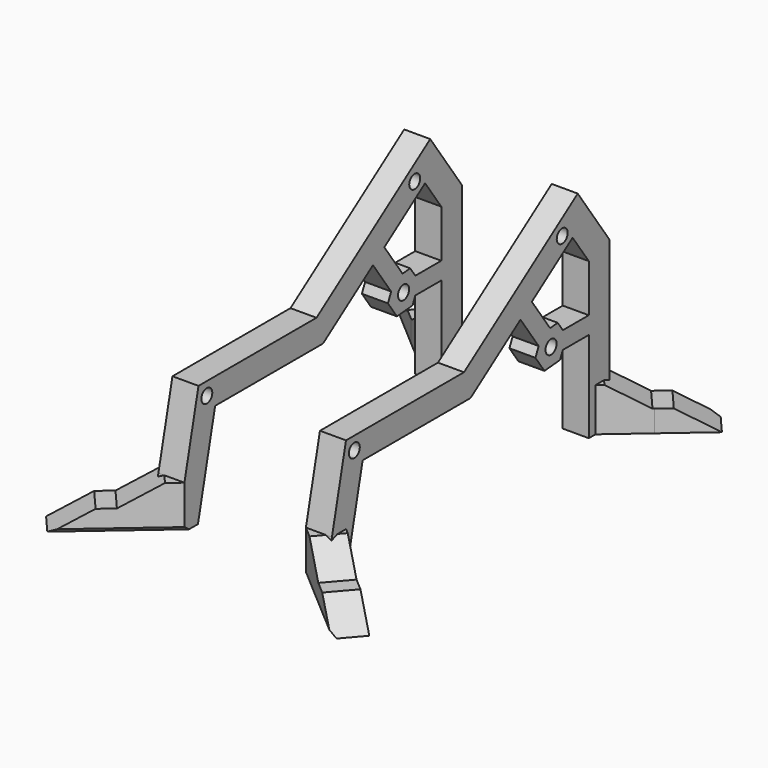
from build123d import *

# Parameters (mm, degrees)
F1_DEPTH     = 70
F2_DEPTH     = 10
F3_DEPTH     = 5
F4_R         = 1.6
F4_R_2       = 1.575
F5_DEPTH     = 25
F6_DEPTH     = 5
F7_SIZE      = 1
F8_T1_DEPTH  = 53.5675435836
F8_T6_DEPTH  = 53.5675435836
F8_T13_DEPTH = 53.5675435836
F8_T19_DEPTH = 53.5675435836
F8_T26_DEPTH = 53.5675435836
F8_T33_DEPTH = 53.5675435836
F9_T1_DEPTH  = 53.5675435836
F9_T6_DEPTH  = 53.5675435836
F9_T12_DEPTH = 53.5675435836
F9_T19_DEPTH = 53.5675435836
F9_T26_DEPTH = 53.5675435836
F9_T32_DEPTH = 53.5675435836


# Not quite as in the source:
# - a fillet or chamfer that OpenCascade refuses, or shapes differently, is made with other operations: its cross-section is extruded or revolved along the edge and cut away or added


with BuildPart() as f1:
    # F0 (on Top) → F1 (new body)
    with BuildSketch(Plane.XY):
        with BuildLine():
            Line((17.481584177, 40), (14, 40))
            Line((14, 40), (18.5698965916, 34.6975434805))
            Line((18.5698965916, 34.6975434805), (20, 35.9300712093))
            Line((20, 35.9300712093), (20, 38.5762325992))
            ThreePointArc((20, 38.5762325992), (18.1979669018, 38.327945742), (17.481584177, 40))
        make_face()
        with BuildLine():
            Line((20, 40), (17.481584177, 40))
            ThreePointArc((17.481584177, 40), (18.1979669018, 38.327945742), (20, 38.5762325992))
            Line((20, 38.5762325992), (20, 40))
        make_face()
        Polygon((18.5698965916, 34.6975434805), (14, 40), (14, 0), (14, -40), (18.5698965916, -34.6975434805), (20, -35.9300712093), (20, 0), (20, 35.9300712093), align=None)
        with BuildLine():
            Line((18.5698965916, -34.6975434805), (14, -40))
            Line((14, -40), (17.481584177, -40))
            ThreePointArc((17.481584177, -40), (18.1979669018, -38.327945742), (20, -38.5762325992))
            Line((20, -38.5762325992), (20, -35.9300712093))
            Line((20, -35.9300712093), (18.5698965916, -34.6975434805))
        make_face()
        with BuildLine():
            ThreePointArc((20, -38.5762325992), (18.1979669018, -38.327945742), (17.481584177, -40))
            Line((17.481584177, -40), (20, -40))
            Line((20, -40), (20, -38.5762325992))
        make_face()
    extrude(amount=F1_DEPTH)

    # F0 (on Top) → F2 (join)
    with BuildSketch(Plane.XY):
        with BuildLine():
            ThreePointArc((20.4361765556, 39.633720036), (19.1207184642, 41.1223248473), (17.481584177, 40))
            Line((17.481584177, 40), (20, 40))
            Line((20, 40), (20, 38.5762325992))
            ThreePointArc((20, 38.5762325992), (20.3228515656, 39.0617651281), (20.4361765556, 39.633720036))
        make_face()
        with BuildLine():
            Line((23.4686723563, 48.1605296279), (14, 40))
            Line((14, 40), (17.481584177, 40))
            ThreePointArc((17.481584177, 40), (19.1207184642, 41.1223248473), (20.4361765556, 39.633720036))
            ThreePointArc((20.4361765556, 39.633720036), (20.3228515656, 39.0617651281), (20, 38.5762325992))
            Line((20, 38.5762325992), (20, 35.9300712093))
            Line((20, 35.9300712093), (28.038568948, 42.8580731084))
            Line((28.038568948, 42.8580731084), (23.4686723563, 48.1605296279))
        make_face()
        with BuildLine():
            Line((17.481584177, -40), (14, -40))
            Line((14, -40), (23.4686723563, -48.1605296279))
            Line((23.4686723563, -48.1605296279), (28.038568948, -42.8580731084))
            Line((28.038568948, -42.8580731084), (20, -35.9300712093))
            Line((20, -35.9300712093), (20, -38.5762325992))
            ThreePointArc((20, -38.5762325992), (20.3228515656, -39.0617651281), (20.4361765556, -39.633720036))
            ThreePointArc((20.4361765556, -39.633720036), (19.1207184642, -41.1223248473), (17.481584177, -40))
        make_face()
        with BuildLine():
            Line((20, -40), (17.481584177, -40))
            ThreePointArc((17.481584177, -40), (19.1207184642, -41.1223248473), (20.4361765556, -39.633720036))
            ThreePointArc((20.4361765556, -39.633720036), (20.3228515656, -39.0617651281), (20, -38.5762325992))
            Line((20, -38.5762325992), (20, -40))
        make_face()
    extrude(amount=F2_DEPTH)

    # F0 (on Top) → F3 (join)
    with BuildSketch(Plane.XY):
        Polygon((32.9373447127, 56.3210592559), (23.4686723563, 48.1605296279), (28.038568948, 42.8580731084), (37.5072413043, 51.0186027363), align=None)
        Polygon((28.038568948, -42.8580731084), (23.4686723563, -48.1605296279), (32.9373447127, -56.3210592559), (37.5072413043, -51.0186027363), align=None)
    extrude(amount=F3_DEPTH)

    # F4 (on face) → F5 (cut)
    with BuildSketch(Plane(origin=(14, 0, 0), x_dir=(0, -1, 0), z_dir=(-1, 0, 0))):
        Polygon((-34, 0), (36.0994255375, 0), (31.1508810268, 22), (0.0593981216, 22), (-14.3160304975, 32.0657834841), (-19.5621121893, 24.5736023727), (-18.6246911161, 22.5632963938), (-21.2215746664, 18.8545623277), (-25.7318743586, 19.2491624199), (-26.5286701393, 20.9578964859), (-34, 20.9578964859), align=None)
        Polygon((-30.8148909167, 50.943057454), (1.9511908549, 28), (35.9511908549, 28), (40, 10), (40, 70), (-40, 70), (-40, 37.825362225), align=None)
        Polygon((-34, 24.9578964859), (-26.5211773832, 24.9578964859), (-25.0484069503, 27.0612306442), (-22.8387203665, 26.8679081181), (-17.5926386747, 34.3600892295), (-29.3414372691, 42.5866865702), (-34, 35.9335694917), align=None)
        with Locations((-23.1349908083, 22.9578964859)):
            Circle(F4_R)
        with Locations((-26.3438594686, 44.1500837642)):
            Circle(F4_R_2)
        with Locations((33.5510359408, 25)):
            Circle(F4_R_2)
    extrude(amount=-F5_DEPTH, mode=Mode.SUBTRACT)

    # F0 (on Top) → F6 (cut)
    with BuildSketch(Plane.XY):
        with BuildLine():
            Line((20, -40), (17.481584177, -40))
            ThreePointArc((17.481584177, -40), (19.1207184642, -41.1223248473), (20.4361765556, -39.633720036))
            ThreePointArc((20.4361765556, -39.633720036), (20.3228515656, -39.0617651281), (20, -38.5762325992))
            Line((20, -38.5762325992), (20, -40))
        make_face()
        with BuildLine():
            ThreePointArc((20, -38.5762325992), (18.1979669018, -38.327945742), (17.481584177, -40))
            Line((17.481584177, -40), (20, -40))
            Line((20, -40), (20, -38.5762325992))
        make_face()
        with BuildLine():
            ThreePointArc((20.4361765556, 39.633720036), (19.1207184642, 41.1223248473), (17.481584177, 40))
            Line((17.481584177, 40), (20, 40))
            Line((20, 40), (20, 38.5762325992))
            ThreePointArc((20, 38.5762325992), (20.3228515656, 39.0617651281), (20.4361765556, 39.633720036))
        make_face()
        with BuildLine():
            Line((20, 40), (17.481584177, 40))
            ThreePointArc((17.481584177, 40), (18.1979669018, 38.327945742), (20, 38.5762325992))
            Line((20, 38.5762325992), (20, 40))
        make_face()
    extrude(amount=F6_DEPTH, mode=Mode.SUBTRACT)

    # F7
    f7_edges = [f1.edges().sort_by_distance(p)[0] for p in [
        (23.468672, -48.16053, 0),
        (23.468672, 48.16053, 0),
    ]]
    chamfer(f7_edges, length=F7_SIZE)

    # F8: chamfer of 9 x 5.1961524227 on 2 edges, made by hand

    # F8_s2 → F8_t1 (cut)
    with BuildSketch(Plane(origin=(-29.0147501324, -33.6658495258, 0), x_dir=(0, 0, 1), z_dir=(0.6528423702, 0.7574937885, 0))):
        Polygon((-0.1961524227, 61.7186078485), (5, 52.7186078485), (5, 61.7186078485), align=None)
    extrude(amount=F8_T1_DEPTH, mode=Mode.SUBTRACT)


with BuildPart() as f8_tool4:
    # F8_s5 → F8_t6 (new body)
    with BuildSketch(Plane(origin=(-29.0147501324, -33.6658495258, 0), x_dir=(0, 0, 1), z_dir=(0.6528423702, 0.7574937885, 0))):
        Polygon((10, 40.2186078485), (4.8038475773, 49.2186078485), (10, 49.2186078485), align=None)
    extrude(amount=F8_T6_DEPTH)

    split(bisect_by=Plane(origin=(0, -40.2146679203, 9.0456397358), x_dir=(1, 0, 0), z_dir=(0, -0.9756235772, 0.219450759)), keep=Keep.TOP)

    split(bisect_by=Plane.YZ.offset(20), keep=Keep.BOTTOM)

    split(bisect_by=Plane.XY.offset(5), keep=Keep.TOP)


with BuildPart() as f1_1:
    add(f1.part)

    # F8_t3: cut F8_tool4
    add(f8_tool4.part, mode=Mode.SUBTRACT)


with BuildPart() as f8_tool11:
    # F8_s12 → F8_t13 (new body)
    with BuildSketch(Plane(origin=(-29.0147501324, -33.6658495258, 0), x_dir=(0, 0, 1), z_dir=(0.6528423702, 0.7574937885, 0))):
        Polygon((10, 40.2186078485), (4.8038475773, 49.2186078485), (10, 49.2186078485), align=None)
    extrude(amount=F8_T13_DEPTH)

    split(bisect_by=Plane.YZ.offset(20), keep=Keep.BOTTOM)

    split(bisect_by=Plane.XY.offset(5), keep=Keep.BOTTOM)


with BuildPart() as f1_2:
    add(f1_1.part)

    # F8_t10: cut F8_tool11
    add(f8_tool11.part, mode=Mode.SUBTRACT)


with BuildPart() as f8_tool17:
    # F8_s18 → F8_t19 (new body)
    with BuildSketch(Plane(origin=(-29.0147501324, -33.6658495258, 0), x_dir=(0, 0, 1), z_dir=(0.6528423702, 0.7574937885, 0))):
        Polygon((10, 40.2186078485), (4.8038475773, 49.2186078485), (10, 49.2186078485), align=None)
    extrude(amount=F8_T19_DEPTH)

    split(bisect_by=Plane(origin=(0, -40.2146679203, 9.0456397358), x_dir=(1, 0, 0), z_dir=(0, -0.9756235772, 0.219450759)), keep=Keep.TOP)

    split(bisect_by=Plane.YZ.offset(20), keep=Keep.TOP)

    split(bisect_by=Plane.XY.offset(5), keep=Keep.TOP)


with BuildPart() as f1_3:
    add(f1_2.part)

    # F8_t16: cut F8_tool17
    add(f8_tool17.part, mode=Mode.SUBTRACT)


with BuildPart() as f8_tool24:
    # F8_s25 → F8_t26 (new body)
    with BuildSketch(Plane(origin=(-29.0147501324, -33.6658495258, 0), x_dir=(0, 0, 1), z_dir=(0.6528423702, 0.7574937885, 0))):
        Polygon((10, 40.2186078485), (4.8038475773, 49.2186078485), (10, 49.2186078485), align=None)
    extrude(amount=F8_T26_DEPTH)

    split(bisect_by=Plane(origin=(0, -40.2146679203, 9.0456397358), x_dir=(1, 0, 0), z_dir=(0, 0.9756235772, -0.219450759)), keep=Keep.TOP)

    split(bisect_by=Plane.YZ.offset(20), keep=Keep.TOP)

    split(bisect_by=Plane.XY.offset(5), keep=Keep.TOP)


with BuildPart() as f1_4:
    add(f1_3.part)

    # F8_t23: cut F8_tool24
    add(f8_tool24.part, mode=Mode.SUBTRACT)


with BuildPart() as f8_tool31:
    # F8_s32 → F8_t33 (new body)
    with BuildSketch(Plane(origin=(-29.0147501324, -33.6658495258, 0), x_dir=(0, 0, 1), z_dir=(0.6528423702, 0.7574937885, 0))):
        Polygon((10, 40.2186078485), (4.8038475773, 49.2186078485), (10, 49.2186078485), align=None)
    extrude(amount=F8_T33_DEPTH)

    split(bisect_by=Plane(origin=(0, -40.2146679203, 9.0456397358), x_dir=(1, 0, 0), z_dir=(0, 0.9756235772, -0.219450759)), keep=Keep.TOP)

    split(bisect_by=Plane.XY.offset(5), keep=Keep.BOTTOM)


with BuildPart() as f1_5:
    add(f1_4.part)

    # F8_t30: cut F8_tool31
    add(f8_tool31.part, mode=Mode.SUBTRACT)

    # F9: chamfer of 9 x 5.1961524227 on 2 edges, made by hand

    # F9_s2 → F9_t1 (cut)
    with BuildSketch(Plane(origin=(5.9564119884, -6.9112320044, 0), x_dir=(0, 0, 1), z_dir=(-0.6528423702, 0.7574937885, 0))):
        Polygon((-0.1961524227, 61.7186078485), (5, 52.7186078485), (5, 61.7186078485), align=None)
    extrude(amount=F9_T1_DEPTH, mode=Mode.SUBTRACT)


with BuildPart() as f9_tool4:
    # F9_s5 → F9_t6 (new body)
    with BuildSketch(Plane(origin=(5.9564119884, -6.9112320044, 0), x_dir=(0, 0, 1), z_dir=(-0.6528423702, 0.7574937885, 0))):
        Polygon((4.8038475773, 49.2186078485), (10, 40.2186078485), (10, 49.2186078485), align=None)
    extrude(amount=F9_T6_DEPTH)

    split(bisect_by=Plane.XY.offset(5), keep=Keep.BOTTOM)

    split(bisect_by=Plane.XZ.offset(-40), keep=Keep.TOP)


with BuildPart() as f1_6:
    add(f1_5.part)

    # F9_t3: cut F9_tool4
    add(f9_tool4.part, mode=Mode.SUBTRACT)


with BuildPart() as f9_tool10:
    # F9_s11 → F9_t12 (new body)
    with BuildSketch(Plane(origin=(5.9564119884, -6.9112320044, 0), x_dir=(0, 0, 1), z_dir=(-0.6528423702, 0.7574937885, 0))):
        Polygon((4.8038475773, 49.2186078485), (10, 40.2186078485), (10, 49.2186078485), align=None)
    extrude(amount=F9_T12_DEPTH)

    split(bisect_by=Plane.YZ.offset(20), keep=Keep.TOP)

    split(bisect_by=Plane.XY.offset(5), keep=Keep.TOP)

    split(bisect_by=Plane.XZ.offset(-40), keep=Keep.TOP)


with BuildPart() as f1_7:
    add(f1_6.part)

    # F9_t9: cut F9_tool10
    add(f9_tool10.part, mode=Mode.SUBTRACT)


with BuildPart() as f9_tool17:
    # F9_s18 → F9_t19 (new body)
    with BuildSketch(Plane(origin=(5.9564119884, -6.9112320044, 0), x_dir=(0, 0, 1), z_dir=(-0.6528423702, 0.7574937885, 0))):
        Polygon((4.8038475773, 49.2186078485), (10, 40.2186078485), (10, 49.2186078485), align=None)
    extrude(amount=F9_T19_DEPTH)

    split(bisect_by=Plane.YZ.offset(20), keep=Keep.TOP)

    split(bisect_by=Plane.XY.offset(5), keep=Keep.TOP)

    split(bisect_by=Plane.XZ.offset(-40), keep=Keep.BOTTOM)


with BuildPart() as f1_8:
    add(f1_7.part)

    # F9_t16: cut F9_tool17
    add(f9_tool17.part, mode=Mode.SUBTRACT)


with BuildPart() as f9_tool24:
    # F9_s25 → F9_t26 (new body)
    with BuildSketch(Plane(origin=(5.9564119884, -6.9112320044, 0), x_dir=(0, 0, 1), z_dir=(-0.6528423702, 0.7574937885, 0))):
        Polygon((4.8038475773, 49.2186078485), (10, 40.2186078485), (10, 49.2186078485), align=None)
    extrude(amount=F9_T26_DEPTH)

    split(bisect_by=Plane.YZ.offset(20), keep=Keep.BOTTOM)

    split(bisect_by=Plane.XY.offset(5), keep=Keep.BOTTOM)


with BuildPart() as f1_9:
    add(f1_8.part)

    # F9_t23: cut F9_tool24
    add(f9_tool24.part, mode=Mode.SUBTRACT)


with BuildPart() as f9_tool30:
    # F9_s31 → F9_t32 (new body)
    with BuildSketch(Plane(origin=(5.9564119884, -6.9112320044, 0), x_dir=(0, 0, 1), z_dir=(-0.6528423702, 0.7574937885, 0))):
        Polygon((4.8038475773, 49.2186078485), (10, 40.2186078485), (10, 49.2186078485), align=None)
    extrude(amount=F9_T32_DEPTH)

    split(bisect_by=Plane.YZ.offset(20), keep=Keep.BOTTOM)

    split(bisect_by=Plane.XY.offset(5), keep=Keep.TOP)

    split(bisect_by=Plane.XZ.offset(-40), keep=Keep.BOTTOM)


with BuildPart() as f1_10:
    add(f1_9.part)

    # F9_t29: cut F9_tool30
    add(f9_tool30.part, mode=Mode.SUBTRACT)


with BuildPart() as f10_1:
    # F10: instance of F1
    add(f1_10.part.mirror(Plane.YZ))


solid = Compound([f1_10.part, f10_1.part])
